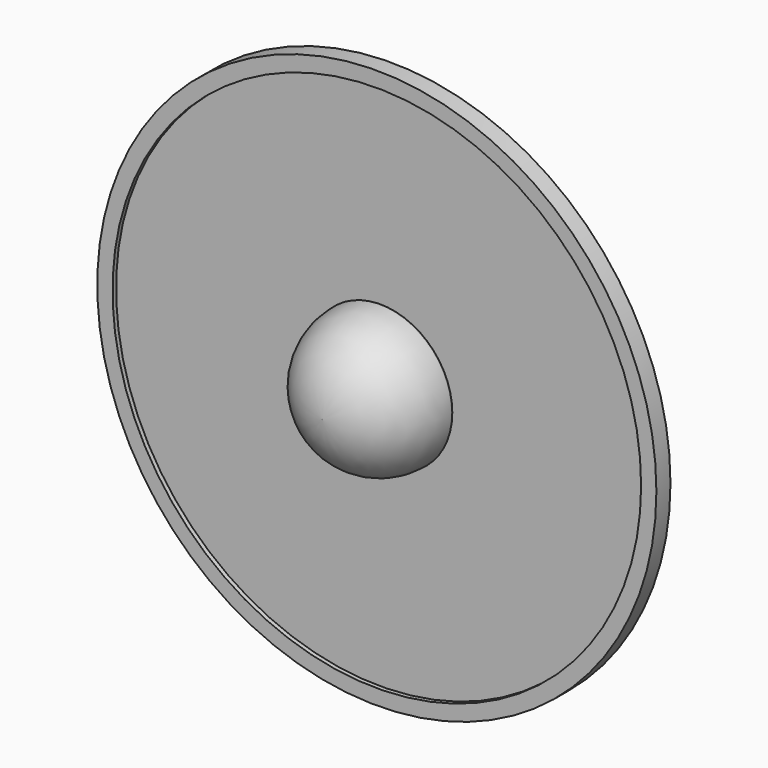
from build123d import *

# Parameters (mm, degrees)
F0_R      = 64.5594783813
F1_DEPTH  = 1.524
F2_R      = 64.5594783813
F2_R_2    = 61.0323113023
F3_DEPTH  = 1.016
F4_R      = 16.6175214607
F5_DEPTH  = 16.764
F6_R      = 16.5608
F7_R      = 61.0868628562
F8_DEPTH  = 1.016
F13_W     = 3.8755843416
F13_H     = 16.3549613208
F13_W_2   = 3.6430479959
F14_DEPTH = 11.7094
F15_W     = 10.4532966083
F15_H     = 12.4406219693
F16_DEPTH = 37.6174


# Not quite as in the source:
# - the program builds the solid bodies; features that only make, move or delete a surface that nothing else refers to are left out


with BuildPart() as f1:
    # F0 (on Front) → F1 (new body, symmetric)
    with BuildSketch(Plane.XZ):
        Circle(F0_R)
    extrude(amount=F1_DEPTH, both=True)

    # F2 (on face) → F3 (join)
    with BuildSketch(Plane.XZ.offset(1.524)):
        Circle(F2_R)
        Circle(F2_R_2, mode=Mode.SUBTRACT)
    extrude(amount=F3_DEPTH)

    # F4 (on face) → F5 (join)
    with BuildSketch(Plane.XZ.offset(1.524)):
        Circle(F4_R)
    extrude(amount=F5_DEPTH)

    # F6
    f6_edges = [f1.edges().sort_by_distance(p)[0] for p in [
        (-16.617521, -18.288, 0),
    ]]
    fillet(f6_edges, radius=F6_R)

    # F7 (on face) → F8 (join)
    with BuildSketch(Plane(origin=(0, 1.524, 0), x_dir=(-1, 0, 0), z_dir=(0, 1, 0))):
        Circle(F7_R)
    extrude(amount=F8_DEPTH)

    # F13 (on face) → F14 (join)
    with BuildSketch(Plane(origin=(0, 2.54, 0), x_dir=(-1, 0, 0), z_dir=(0, 1, 0))):
        with Locations((-13.9141972177, -4.206892103)):
            Rectangle(F13_W, F13_H)
        with Locations((16.1215732805, -4.206892103)):
            Rectangle(F13_W_2, F13_H)
    extrude(amount=F14_DEPTH)

    # F15 (on face) → F16 (cut)
    with BuildSketch(Plane(origin=(-17.9430972785, 0, 0), x_dir=(0, -1, 0), z_dir=(-1, 0, 0))):
        with Locations((-7.7666483042, -4.7159082606)):
            Rectangle(F15_W, F15_H)
    extrude(amount=-F16_DEPTH, mode=Mode.SUBTRACT)


solid = f1.part
